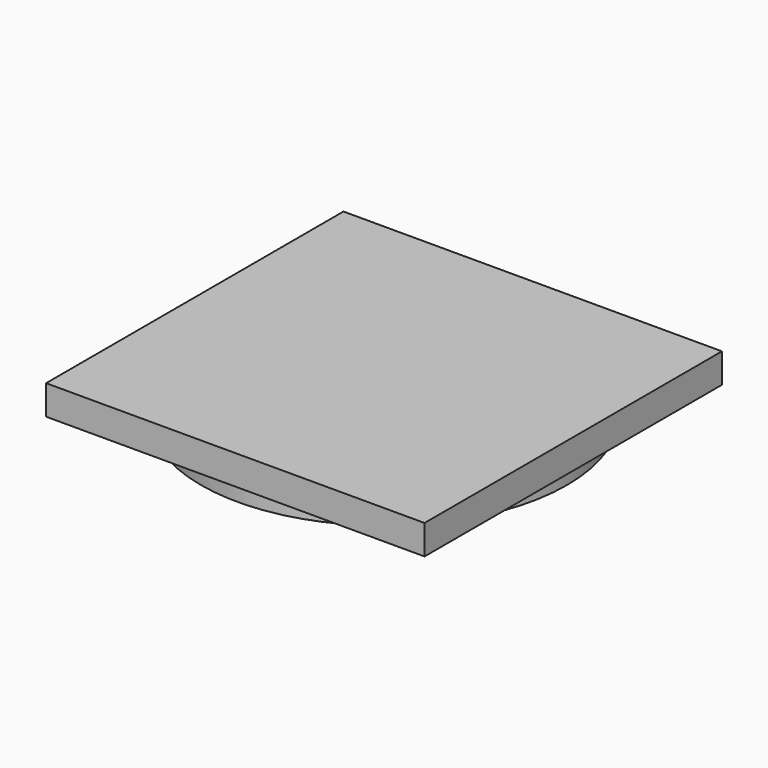
from build123d import *

# Parameters (mm, degrees)
F1_START        = -50.8
F0_R            = 314.96
F0_R_2          = 31.75
F1_DEPTH        = 50.8
F3_DEPTH        = 314.96
F3_COPIES_COUNT = 3
F3_COPIES_ANGLE = 120
F5_START        = -25.4
F4_W            = 651.5112519264
F4_H            = 639.9160027504
F5_DEPTH        = 50.8


# Not quite as in the source:
# - a pattern or mirror of a feature is missing from the dataset's text; its kind, count and spacing are read off the source's solid


with BuildPart() as f1:
    # F0 (on Top) → F1 (new body)
    with BuildSketch(Plane.XY.offset(F1_START)):
        Circle(F0_R)
        Circle(F0_R_2, mode=Mode.SUBTRACT)
    extrude(amount=-F1_DEPTH)

    # F2 (on Front) → F3 (cut, symmetric)
    with BuildSketch(Plane.XZ):
        Polygon((7.9375, -50.8), (0, -50.8), (-7.9375, -50.8), (-7.9375, -66.675), (-12.7, -66.675), (-12.7, -79.375), (0, -79.375), (12.7, -79.375), (12.7, -66.675), (7.9375, -66.675), align=None)
    f3 = extrude(amount=F3_DEPTH, both=True, mode=Mode.SUBTRACT)

    # F3_copies: F3 ×3 about axis
    f3_copies_axis = Axis((0, 0, 0), (0, 0, 1))
    for i in range(1, F3_COPIES_COUNT):
        add(f3.rotate(f3_copies_axis, i * F3_COPIES_ANGLE / (F3_COPIES_COUNT - 1)), mode=Mode.SUBTRACT)


with BuildPart() as f5:
    # F4 (on Top) → F5 (new body)
    with BuildSketch(Plane.XY.offset(F5_START)):
        Rectangle(F4_W, F4_H)
    extrude(amount=-F5_DEPTH)


solid = Compound([f1.part, f5.part])
